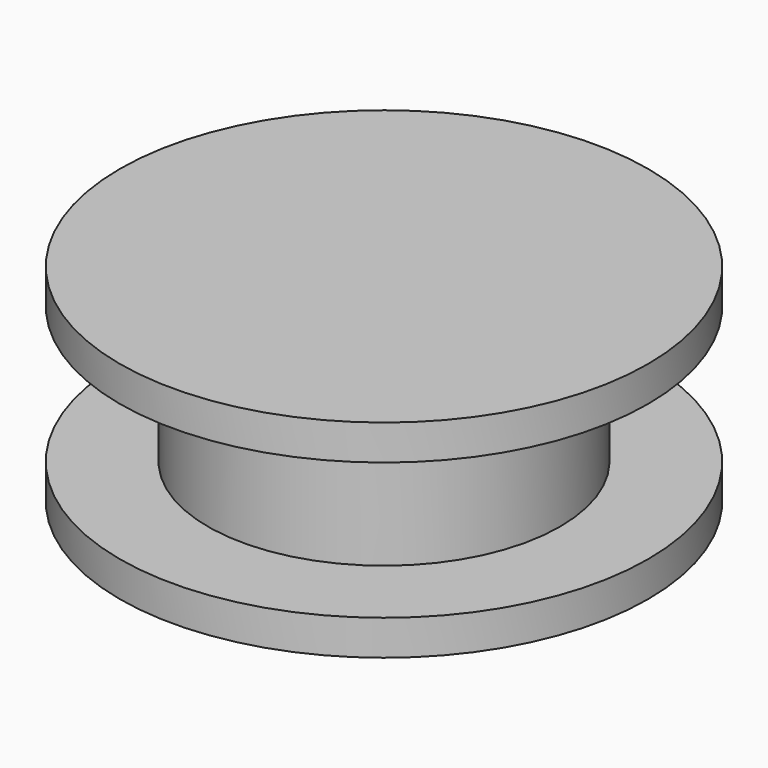
from build123d import *

# Parameters (mm, degrees)
F0_R     = 1
F1_DEPTH = 0.776
F2_R     = 1.5
F2_R_2   = 1
F3_DEPTH = 0.2
F4_R     = 1.5
F4_R_2   = 1
F5_DEPTH = 0.2


with BuildPart() as f1:
    # F0 (on Top) → F1 (new body)
    with BuildSketch(Plane.XY):
        Circle(F0_R)
    extrude(amount=F1_DEPTH)

    # F2 (on face) → F3 (join)
    with BuildSketch(Plane.XY.offset(0.776)):
        Circle(F2_R)
        Circle(F2_R_2, mode=Mode.SUBTRACT)
        Circle(F2_R_2)
    extrude(amount=F3_DEPTH)

    # F4 (on face) → F5 (join)
    with BuildSketch(Plane(origin=(0, 0, 0), x_dir=(1, 0, 0), z_dir=(0, 0, -1))):
        Circle(F4_R)
        Circle(F4_R_2, mode=Mode.SUBTRACT)
        Circle(F4_R_2)
    extrude(amount=F5_DEPTH)


solid = f1.part
